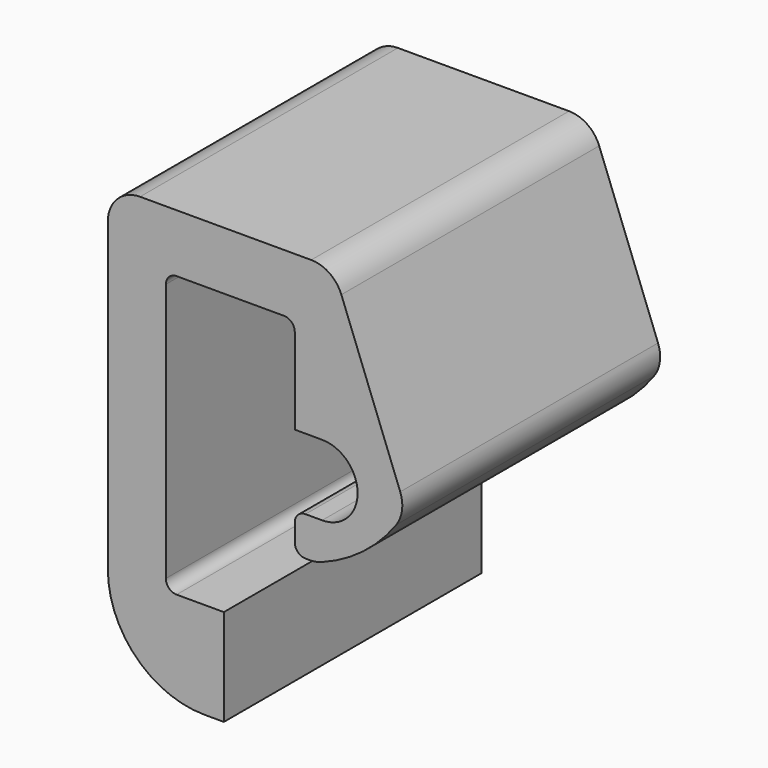
from build123d import *

# Parameters (mm, degrees)
F1_DEPTH = 10
F2_R     = 1
F3_R     = 3
F4_R     = 0.33333


with BuildPart() as f1:
    # F0 (on Front) → F1 (new body)
    with BuildSketch(Plane.XZ):
        with BuildLine():
            Line((0, 0), (3.6, 0))
            Line((3.6, 0), (3.6, 3))
            Line((3.6, 3), (1.8, 3))
            Line((1.8, 3), (1.8, 11.7))
            Line((1.8, 11.7), (5.8, 11.7))
            Line((5.8, 11.7), (5.8, 8.7))
            Line((5.8, 8.7), (6.6518087818, 8.6985993288))
            ThreePointArc((6.6518087818, 8.6985993288), (7.4284566976, 8.3757785113), (7.75, 7.598600816))
            Line((7.75, 7.598600816), (9.25, 7.598600816))
            Line((9.25, 7.598600816), (7, 13.5))
            Line((7, 13.5), (0, 13.5))
            Line((0, 13.5), (0, 0))
        make_face()
        with BuildLine():
            ThreePointArc((6.4457045279, 5.2862485499), (8.0654097754, 6.1785827272), (9.25, 7.598600816))
            Line((9.25, 7.598600816), (7.75, 7.598600816))
            ThreePointArc((7.75, 7.598600816), (7.4278174593, 6.8207833567), (6.65, 6.498600816))
            Line((6.65, 6.498600816), (5.8, 6.498600816))
            Line((5.8, 6.498600816), (5.8, 5.2862485499))
            Line((5.8, 5.2862485499), (6.4457045279, 5.2862485499))
        make_face()
    extrude(amount=F1_DEPTH)

    # F2
    f2_edges = [f1.edges().sort_by_distance(p)[0] for p in [
        (0, -5, 13.5),
        (7, -5, 13.5),
        (6.445705, -5, 5.286249),
        (9.25, -5, 7.598601),
    ]]
    fillet(f2_edges, radius=F2_R)

    # F3
    f3_edges = [f1.edges().sort_by_distance(p)[0] for p in [
        (0, -5, 0),
    ]]
    fillet(f3_edges, radius=F3_R)

    # F4
    f4_edges = [f1.edges().sort_by_distance(p)[0] for p in [
        (5.8, -5, 11.7),
        (5.8, -5, 5.286249),
        (5.8, -5, 6.498601),
        (1.8, -5, 3),
        (1.8, -5, 11.7),
    ]]
    fillet(f4_edges, radius=F4_R)


solid = f1.part
